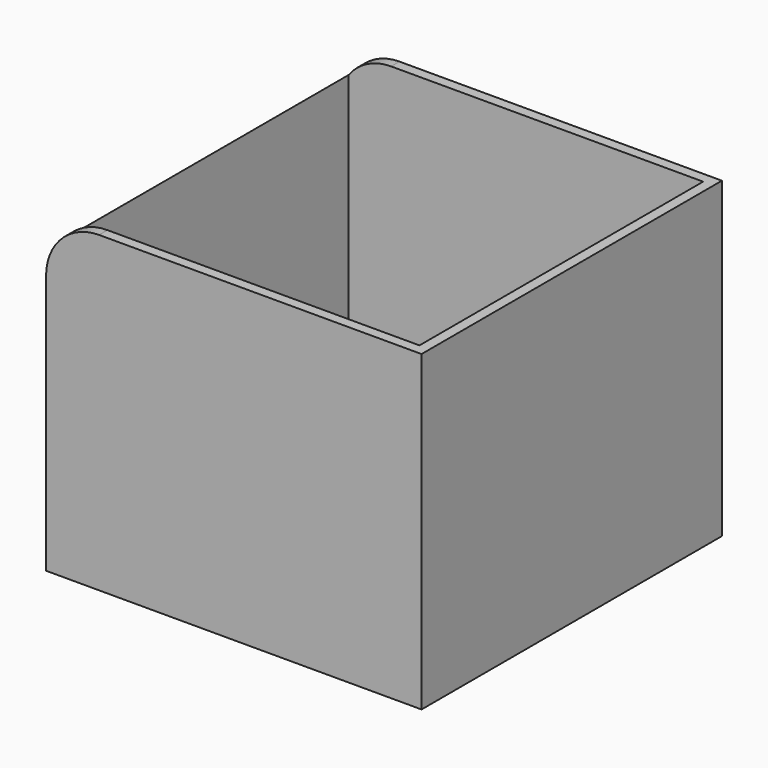
from build123d import *

# Parameters (mm, degrees)
F0_W        = 72
F0_H        = 72
F1_DEPTH    = 60
F2_W        = 68
F2_H        = 68
F3_DEPTH    = 58
F4_T1_DEPTH = 122.8


# Not quite as in the source:
# - a fillet or chamfer that OpenCascade refuses, or shapes differently, is made with other operations: its cross-section is extruded or revolved along the edge and cut away or added


with BuildPart() as f1:
    # F0 (on Top) → F1 (new body)
    with BuildSketch(Plane.XY):
        with Locations((24.6826619834, 21.6548714693)):
            Rectangle(F0_W, F0_H)
    extrude(amount=F1_DEPTH)

    # F2 (on face) → F3 (cut)
    with BuildSketch(Plane.XY.offset(60)):
        with Locations((24.6826619834, 21.6548714693)):
            Rectangle(F2_W, F2_H)
    extrude(amount=-F3_DEPTH, mode=Mode.SUBTRACT)

    # F4: fillet of radius 10.16 on 1 edges, made by hand

    # F4_s2 → F4_t1 (cut)
    with BuildSketch(Plane.XZ.offset(-83.0548714693)):
        with BuildLine():
            ThreePointArc((-1.1573380166, 60), (-8.3415429135, 57.0242048969), (-11.3173380166, 49.84))
            Line((-11.3173380166, 49.84), (-11.3173380166, 60))
            Line((-11.3173380166, 60), (-1.1573380166, 60))
        make_face()
    extrude(amount=F4_T1_DEPTH, mode=Mode.SUBTRACT)


solid = f1.part
